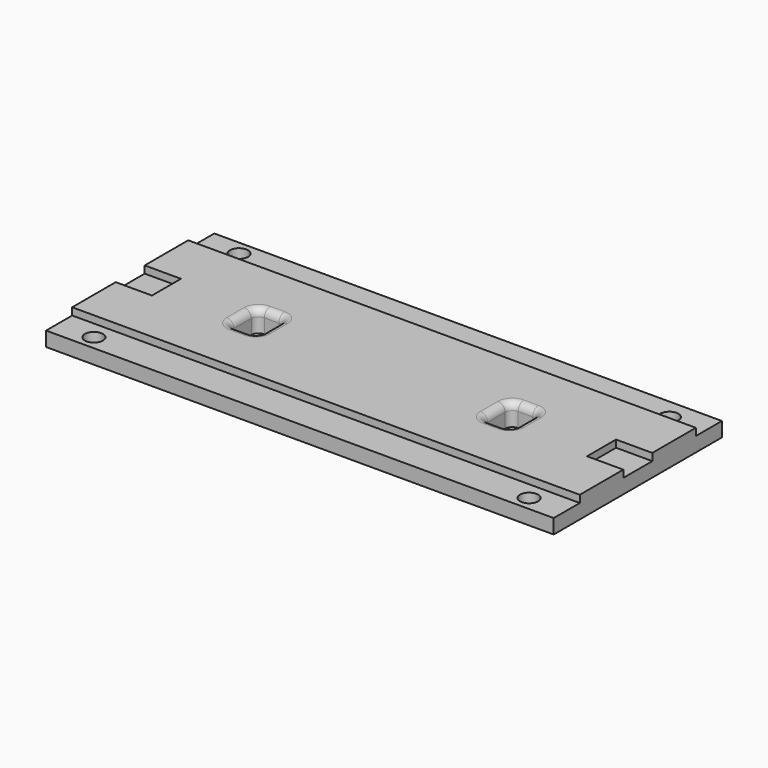
from build123d import *

# Parameters (mm, degrees)
F0_W     = 4
F0_H     = 5
F1_DEPTH = 3
F0_W_2   = 5
F0_W_3   = 70
F0_H_2   = 4.5
F2_DEPTH = 2
F3_D     = 2.5
F4_F1_R  = 1
F4_F2_R  = 1


with BuildPart() as f1:
    # F0 (on Top) → F1 (new body)
    with BuildSketch(Plane.XY):
        Polygon((-35, -10), (35, -10), (35, -2.5), (30, -2.5), (30, 2.5), (35, 2.5), (35, 10), (-35, 10), (-35, 2.5), (-30, 2.5), (-30, -2.5), (-35, -2.5), align=None)
        with Locations((-17.5, 0)):
            Rectangle(F0_W, F0_H, mode=Mode.SUBTRACT)
        with Locations((17.5, 0)):
            Rectangle(F0_W, F0_H, mode=Mode.SUBTRACT)
    extrude(amount=F1_DEPTH)

    # F0 (on Top) → F2 (join)
    with BuildSketch(Plane.XY):
        with Locations((-32.5, 0)):
            Rectangle(F0_W_2, F0_H)
        with Locations((0, 12.25)):
            Rectangle(F0_W_3, F0_H_2)
        with Locations((0, -12.25)):
            Rectangle(F0_W_3, F0_H_2)
        with Locations((32.5, 0)):
            Rectangle(F0_W_2, F0_H)
    extrude(amount=F2_DEPTH)

    # F3 (through all)
    with Locations(Plane(origin=(0, 0, 0), x_dir=(1, 0, 0), z_dir=(0, 0, -1))):
        with Locations((-30, 12.5), (-30, -12.5), (30, -11.6784099489), (30, 12.5)):
            Hole(F3_D / 2)

    # F4: fillet of radius 1 on 12 edges, made by hand

    # F4_f1
    f4_f1_edges = [f1.edges().sort_by_distance(p)[0] for p in [
        (-19.5, 2.5, 1.5),
        (-15.5, 2.5, 1.5),
        (-15.5, -2.5, 1.5),
        (-19.5, -2.5, 1.5),
        (19.5, 2.5, 1.5),
        (19.5, -2.5, 1.5),
        (15.5, -2.5, 1.5),
        (15.5, 2.5, 1.5),
    ]]
    fillet(f4_f1_edges, radius=F4_F1_R)

    # F4_f2
    f4_f2_edges = [f1.edges().sort_by_distance(p)[0] for p in [
        (15.5, 0, 3),
        (-15.5, 0, 3),
        (-19.5, 0, 3),
        (19.5, 0, 3),
        (19.2071067812, 2.2071067812, 3),
        (19.2071067812, -2.2071067812, 3),
        (-19.2071067812, -2.2071067812, 3),
        (-19.2071067812, 2.2071067812, 3),
        (-15.7928932188, 2.2071067812, 3),
        (-15.7928932188, -2.2071067812, 3),
        (15.7928932188, -2.2071067812, 3),
        (15.7928932188, 2.2071067812, 3),
    ]]
    fillet(f4_f2_edges, radius=F4_F2_R)


solid = f1.part
